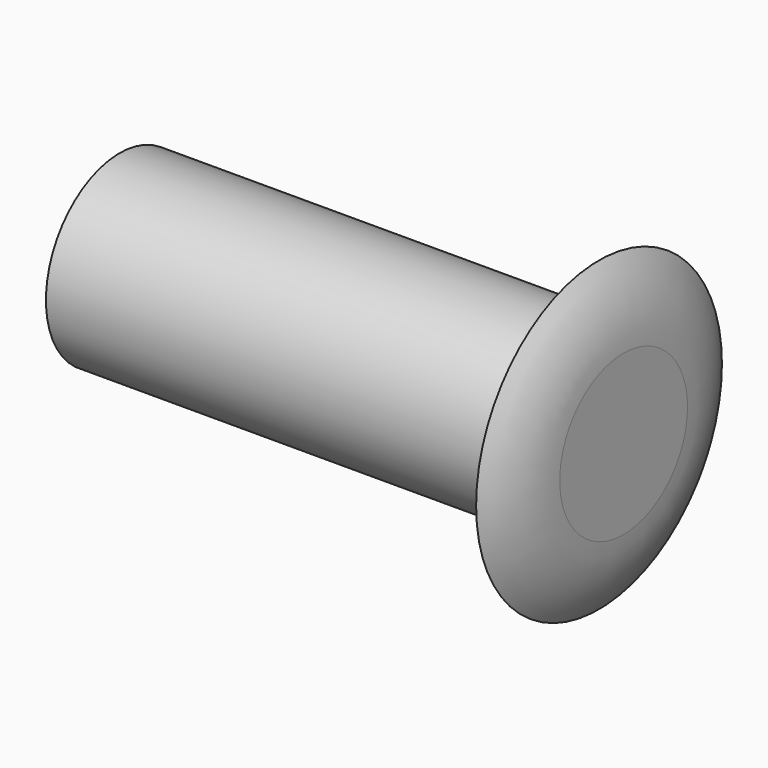
from build123d import *

# Parameters (mm, degrees)
F0_R     = 9.525
F1_DEPTH = 49.53
F2_R     = 15.875
F2_R_2   = 9.525
F3_DEPTH = 2.54


# Not quite as in the source:
# - a fillet or chamfer that OpenCascade refuses, or shapes differently, is made with other operations: its cross-section is extruded or revolved along the edge and cut away or added


with BuildPart() as f1:
    # F0 (on Right) → F1 (new body)
    with BuildSketch(Plane.YZ):
        Circle(F0_R)
    extrude(amount=F1_DEPTH)

    # F2 (on face) → F3 (join)
    with BuildSketch(Plane.YZ.offset(49.53)):
        Circle(F2_R)
        Circle(F2_R_2, mode=Mode.SUBTRACT)
        Circle(F2_R_2)
    extrude(amount=F3_DEPTH)

    # F4: fillet of radius 12.7 on 1 edges, made by hand

    # F4_s1 → F4_t2 (revolve, cut)
    with BuildSketch(Plane.XY):
        with BuildLine():
            ThreePointArc((49.53, 15.875), (51.4182778852, 12.2710926284), (52.07, 8.255))
            Line((52.07, 8.255), (52.07, 15.875))
            Line((52.07, 15.875), (49.53, 15.875))
        make_face()
    revolve(axis=Axis((52.07, 0, 0), (1, 0, 0)), mode=Mode.SUBTRACT)


solid = f1.part
